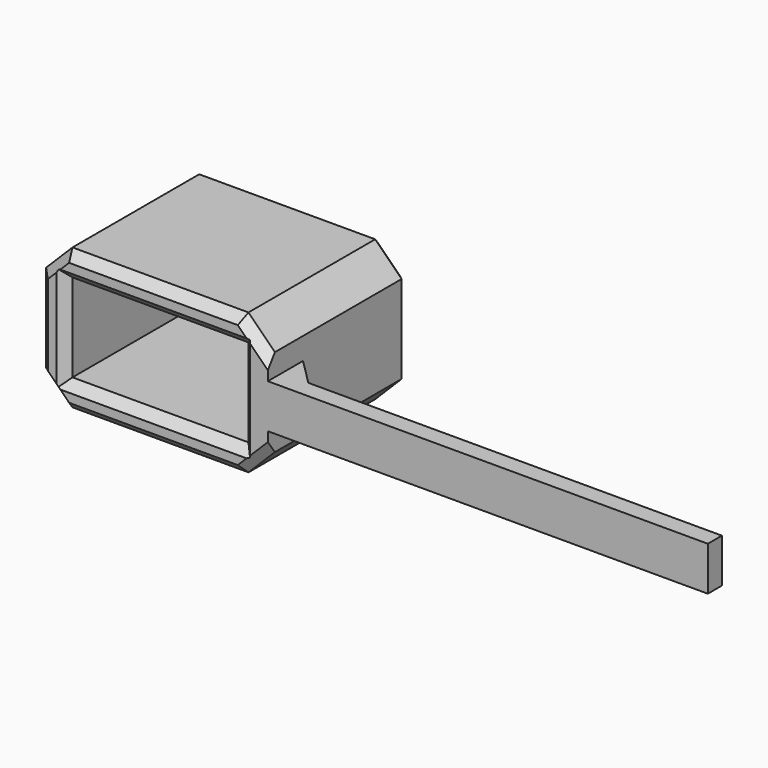
from build123d import *

# Parameters (mm, degrees)
F0_W         = 26
F0_H         = 16
F0_W_2       = 20
F0_H_2       = 10
F1_DEPTH     = 20
F3_DEPTH     = 50
F4_SIZE      = 3
F5_T1_DEPTH  = 10
F5_T3_DEPTH  = 20
F5_T5_DEPTH  = 9.3860066631
F5_T7_DEPTH  = 9.3860066631
F5_T9_DEPTH  = 9.3860066631
F5_T11_DEPTH = 9.3860066631
F5_T13_DEPTH = 25.1433659759
F5_T15_DEPTH = 15.1433659759
F5_T21_DEPTH = 22.571682988
F5_T25_DEPTH = 12.571682988
F5_T32_DEPTH = 22.571682988
F5_T36_DEPTH = 12.571682988
F5_T43_DEPTH = 12.571682988
F5_T47_DEPTH = 22.571682988
F5_T54_DEPTH = 22.571682988
F5_T58_DEPTH = 12.571682988
F6_T1_DEPTH  = 9.3860066631
F6_T3_DEPTH  = 10
F6_T5_DEPTH  = 9.3860066631
F6_T7_DEPTH  = 25.1433659759
F6_T9_DEPTH  = 20
F6_T14_DEPTH = 9.3860066631
F6_T19_DEPTH = 9.3860066631
F6_T25_DEPTH = 22.571682988
F6_T30_DEPTH = 12.571682988
F6_T38_DEPTH = 22.571682988
F6_T43_DEPTH = 12.571682988
F6_T51_DEPTH = 22.571682988
F6_T56_DEPTH = 12.571682988
F6_T64_DEPTH = 12.571682988
F6_T69_DEPTH = 22.571682988
F7_SIZE      = 1


# Not quite as in the source:
# - a fillet or chamfer that OpenCascade refuses, or shapes differently, is made with other operations: its cross-section is extruded or revolved along the edge and cut away or added


with BuildPart() as f1:
    # F0 (on Front) → F1 (new body)
    with BuildSketch(Plane.XZ):
        with Locations((10, 5)):
            Rectangle(F0_W, F0_H)
        with Locations((10, 5)):
            Rectangle(F0_W_2, F0_H_2, mode=Mode.SUBTRACT)
    extrude(amount=F1_DEPTH)

    # F2 (on face) → F3 (join)
    with BuildSketch(Plane.YZ.offset(23)):
        Polygon((-18, 2.5), (-18, 5), (-18, 7.5), (-20, 7.5), (-20, 5), (-20, 2.5), align=None)
    extrude(amount=F3_DEPTH)

    # F4
    f4_edges = [f1.edges().sort_by_distance(p)[0] for p in [
        (-3, -10, 13),
        (23, -10, 13),
        (23, -18, 5),
        (-3, -10, -3),
        (23, -10, -3),
    ]]
    chamfer(f4_edges, length=F4_SIZE)

    # F5: chamfer of 1 on 12 edges, made by hand

    # F5_s2 → F5_t1 (cut)
    with BuildSketch(Plane.XY):
        Polygon((21, 0), (20, -1), (20, 0), align=None)
        Polygon((-1, 0), (0, -1), (0, 0), align=None)
    extrude(amount=F5_T1_DEPTH, mode=Mode.SUBTRACT)

    # F5_s4 → F5_t3 (cut)
    with BuildSketch(Plane.YZ):
        Polygon((0, 11), (-1, 10), (0, 10), align=None)
        Polygon((0, -1), (-1, 0), (0, 0), align=None)
    extrude(amount=F5_T3_DEPTH, mode=Mode.SUBTRACT)

    # F5_s6 → F5_t5 (cut)
    with BuildSketch(Plane(origin=(-3.3184544799, 0, 3.3184544799), x_dir=(0, 1, 0), z_dir=(0.7071067812, 0, -0.7071067812))):
        Polygon((0, -1.1213203436), (-1, -2.1213203436), (0, -2.1213203436), align=None)
    extrude(amount=F5_T5_DEPTH, mode=Mode.SUBTRACT)

    # F5_s8 → F5_t7 (cut)
    with BuildSketch(Plane(origin=(13.3184544799, 0, 13.3184544799), x_dir=(0, 1, 0), z_dir=(-0.7071067812, 0, -0.7071067812))):
        Polygon((0, 15.2634559673), (-1, 16.2634559673), (0, 16.2634559673), align=None)
    extrude(amount=F5_T7_DEPTH, mode=Mode.SUBTRACT)

    # F5_s10 → F5_t9 (cut)
    with BuildSketch(Plane(origin=(1.6815455201, 0, -1.6815455201), x_dir=(0, 1, 0), z_dir=(0.7071067812, 0, -0.7071067812))):
        Polygon((0, 22.3345237792), (-1, 23.3345237792), (0, 23.3345237792), align=None)
    extrude(amount=F5_T9_DEPTH, mode=Mode.SUBTRACT)

    # F5_s12 → F5_t11 (cut)
    with BuildSketch(Plane(origin=(8.3184544799, 0, 8.3184544799), x_dir=(0, 1, 0), z_dir=(-0.7071067812, 0, -0.7071067812))):
        Polygon((0, -8.1923881554), (-1, -9.1923881554), (0, -9.1923881554), align=None)
    extrude(amount=F5_T11_DEPTH, mode=Mode.SUBTRACT)

    # F5_s14 → F5_t13 (cut)
    with BuildSketch(Plane.YZ.offset(-2.571682988)):
        Polygon((0, -2), (-1, -3), (0, -3), align=None)
        Polygon((-1, 13), (0, 12), (0, 13), align=None)
    extrude(amount=F5_T13_DEPTH, mode=Mode.SUBTRACT)

    # F5_s16 → F5_t15 (cut)
    with BuildSketch(Plane.XY.offset(-2.571682988)):
        Polygon((22, 0), (23, -1), (23, 0), align=None)
        Polygon((-2, 0), (-3, -1), (-3, 0), align=None)
    extrude(amount=F5_T15_DEPTH, mode=Mode.SUBTRACT)


with BuildPart() as f5_tool19:
    # F5_s20 → F5_t21 (new body)
    with BuildSketch(Plane.YZ):
        Polygon((0, 11), (-1, 10), (0, 10), align=None)
    extrude(amount=F5_T21_DEPTH)

    split(bisect_by=Plane.YZ.offset(20), keep=Keep.TOP)


with BuildPart() as f5_tool23:
    # F5_s24 → F5_t25 (new body)
    with BuildSketch(Plane.XY.offset(12.571682988)):
        Polygon((21, 0), (20, -1), (20, 0), align=None)
    extrude(amount=-F5_T25_DEPTH)

    split(bisect_by=Plane.XY.offset(10), keep=Keep.TOP)


with BuildPart() as f5_tool19_1:
    add(f5_tool19.part)

    # F5_t27: intersect F5_tool23
    add(f5_tool23.part, mode=Mode.INTERSECT)


with BuildPart() as f1_1:
    add(f1.part)

    # F5_t17: cut F5_tool19
    add(f5_tool19_1.part, mode=Mode.SUBTRACT)


with BuildPart() as f5_tool30:
    # F5_s31 → F5_t32 (new body)
    with BuildSketch(Plane.YZ.offset(22.571682988)):
        Polygon((0, -1), (-1, 0), (0, 0), align=None)
    extrude(amount=-F5_T32_DEPTH)

    split(bisect_by=Plane.YZ.offset(20), keep=Keep.TOP)


with BuildPart() as f5_tool34:
    # F5_s35 → F5_t36 (new body)
    with BuildSketch(Plane.XY.offset(10)):
        Polygon((21, 0), (20, -1), (20, 0), align=None)
    extrude(amount=-F5_T36_DEPTH)

    split(bisect_by=Plane.XY, keep=Keep.BOTTOM)


with BuildPart() as f5_tool30_1:
    add(f5_tool30.part)

    # F5_t38: intersect F5_tool34
    add(f5_tool34.part, mode=Mode.INTERSECT)


with BuildPart() as f1_2:
    add(f1_1.part)

    # F5_t28: cut F5_tool30
    add(f5_tool30_1.part, mode=Mode.SUBTRACT)


with BuildPart() as f5_tool41:
    # F5_s42 → F5_t43 (new body)
    with BuildSketch(Plane.XY):
        Polygon((-1, 0), (0, -1), (0, 0), align=None)
    extrude(amount=F5_T43_DEPTH)

    split(bisect_by=Plane.XY.offset(10), keep=Keep.TOP)


with BuildPart() as f5_tool45:
    # F5_s46 → F5_t47 (new body)
    with BuildSketch(Plane.YZ.offset(-2.571682988)):
        Polygon((0, 11), (-1, 10), (0, 10), align=None)
    extrude(amount=F5_T47_DEPTH)

    split(bisect_by=Plane.YZ, keep=Keep.BOTTOM)


with BuildPart() as f5_tool41_1:
    add(f5_tool41.part)

    # F5_t49: intersect F5_tool45
    add(f5_tool45.part, mode=Mode.INTERSECT)


with BuildPart() as f1_3:
    add(f1_2.part)

    # F5_t39: cut F5_tool41
    add(f5_tool41_1.part, mode=Mode.SUBTRACT)


with BuildPart() as f5_tool52:
    # F5_s53 → F5_t54 (new body)
    with BuildSketch(Plane.YZ.offset(20)):
        Polygon((0, -1), (-1, 0), (0, 0), align=None)
    extrude(amount=-F5_T54_DEPTH)

    split(bisect_by=Plane.YZ, keep=Keep.BOTTOM)


with BuildPart() as f5_tool56:
    # F5_s57 → F5_t58 (new body)
    with BuildSketch(Plane.XY.offset(-2.571682988)):
        Polygon((-1, 0), (0, -1), (0, 0), align=None)
    extrude(amount=F5_T58_DEPTH)

    split(bisect_by=Plane.XY, keep=Keep.BOTTOM)


with BuildPart() as f5_tool52_1:
    add(f5_tool52.part)

    # F5_t60: intersect F5_tool56
    add(f5_tool56.part, mode=Mode.INTERSECT)


with BuildPart() as f1_4:
    add(f1_3.part)

    # F5_t50: cut F5_tool52
    add(f5_tool52_1.part, mode=Mode.SUBTRACT)

    # F6: chamfer of 1 on 10 edges, made by hand

    # F6_s2 → F6_t1 (cut)
    with BuildSketch(Plane(origin=(-3.3184544799, 0, 3.3184544799), x_dir=(0, 1, 0), z_dir=(0.7071067812, 0, -0.7071067812))):
        Polygon((-19, -2.1213203436), (-20, -1.1213203436), (-20, -2.1213203436), align=None)
    extrude(amount=F6_T1_DEPTH, mode=Mode.SUBTRACT)

    # F6_s4 → F6_t3 (cut)
    with BuildSketch(Plane.XY):
        Polygon((0, -19), (-1, -20), (0, -20), align=None)
        Polygon((20, -19), (21, -20), (20, -20), align=None)
    extrude(amount=F6_T3_DEPTH, mode=Mode.SUBTRACT)

    # F6_s6 → F6_t5 (cut)
    with BuildSketch(Plane(origin=(8.3184544799, 0, 8.3184544799), x_dir=(0, 1, 0), z_dir=(-0.7071067812, 0, -0.7071067812))):
        Polygon((-20, -8.1923881554), (-19, -9.1923881554), (-20, -9.1923881554), align=None)
    extrude(amount=F6_T5_DEPTH, mode=Mode.SUBTRACT)

    # F6_s8 → F6_t7 (cut)
    with BuildSketch(Plane.YZ.offset(-2.571682988)):
        Polygon((-19, -3), (-20, -2), (-20, -3), align=None)
        Polygon((-19, 13), (-20, 12), (-20, 13), align=None)
    extrude(amount=F6_T7_DEPTH, mode=Mode.SUBTRACT)

    # F6_s10 → F6_t9 (cut)
    with BuildSketch(Plane.YZ):
        Polygon((-19, 0), (-20, -1), (-20, 0), align=None)
        Polygon((-19, 10), (-20, 11), (-20, 10), align=None)
    extrude(amount=F6_T9_DEPTH, mode=Mode.SUBTRACT)


with BuildPart() as f6_tool12:
    # F6_s13 → F6_t14 (new body)
    with BuildSketch(Plane(origin=(1.6815455201, 0, -1.6815455201), x_dir=(0, 1, 0), z_dir=(0.7071067812, 0, -0.7071067812))):
        Polygon((-19, 23.3345237792), (-20, 22.3345237792), (-20, 23.3345237792), align=None)
    extrude(amount=F6_T14_DEPTH)

    split(bisect_by=Plane.XY.offset(7.5), keep=Keep.TOP)


with BuildPart() as f1_5:
    add(f1_4.part)

    # F6_t11: cut F6_tool12
    add(f6_tool12.part, mode=Mode.SUBTRACT)


with BuildPart() as f6_tool17:
    # F6_s18 → F6_t19 (new body)
    with BuildSketch(Plane(origin=(13.3184544799, 0, 13.3184544799), x_dir=(0, 1, 0), z_dir=(-0.7071067812, 0, -0.7071067812))):
        Polygon((-19, 16.2634559673), (-20, 15.2634559673), (-20, 16.2634559673), align=None)
    extrude(amount=F6_T19_DEPTH)

    split(bisect_by=Plane.XY.offset(2.5), keep=Keep.BOTTOM)


with BuildPart() as f1_6:
    add(f1_5.part)

    # F6_t16: cut F6_tool17
    add(f6_tool17.part, mode=Mode.SUBTRACT)


with BuildPart() as f6_tool23:
    # F6_s24 → F6_t25 (new body)
    with BuildSketch(Plane.YZ.offset(20)):
        Polygon((-19, 0), (-20, -1), (-20, 0), align=None)
    extrude(amount=-F6_T25_DEPTH)

    split(bisect_by=Plane(origin=(-1.5, 0, -1.5), x_dir=(0, 1, 0), z_dir=(0.7071067812, 0, 0.7071067812)), keep=Keep.TOP)

    split(bisect_by=Plane.YZ, keep=Keep.BOTTOM)


with BuildPart() as f6_tool28:
    # F6_s29 → F6_t30 (new body)
    with BuildSketch(Plane.XY.offset(-2.571682988)):
        Polygon((0, -19), (-1, -20), (0, -20), align=None)
    extrude(amount=F6_T30_DEPTH)

    split(bisect_by=Plane(origin=(-1.5, 0, -1.5), x_dir=(0, 1, 0), z_dir=(0.7071067812, 0, 0.7071067812)), keep=Keep.TOP)

    split(bisect_by=Plane.XY, keep=Keep.BOTTOM)


with BuildPart() as f6_tool23_1:
    add(f6_tool23.part)

    # F6_t33: intersect F6_tool28
    add(f6_tool28.part, mode=Mode.INTERSECT)


with BuildPart() as f1_7:
    add(f1_6.part)

    # F6_t21: cut F6_tool23
    add(f6_tool23_1.part, mode=Mode.SUBTRACT)


with BuildPart() as f6_tool36:
    # F6_s37 → F6_t38 (new body)
    with BuildSketch(Plane.YZ.offset(-2.571682988)):
        Polygon((-19, 10), (-20, 11), (-20, 10), align=None)
    extrude(amount=F6_T38_DEPTH)

    split(bisect_by=Plane.YZ, keep=Keep.BOTTOM)

    split(bisect_by=Plane(origin=(-6.5, 0, 6.5), x_dir=(0, 1, 0), z_dir=(0.7071067812, 0, -0.7071067812)), keep=Keep.TOP)


with BuildPart() as f6_tool41:
    # F6_s42 → F6_t43 (new body)
    with BuildSketch(Plane.XY):
        Polygon((0, -19), (-1, -20), (0, -20), align=None)
    extrude(amount=F6_T43_DEPTH)

    split(bisect_by=Plane.XY.offset(10), keep=Keep.TOP)

    split(bisect_by=Plane(origin=(-6.5, 0, 6.5), x_dir=(0, 1, 0), z_dir=(0.7071067812, 0, -0.7071067812)), keep=Keep.TOP)


with BuildPart() as f6_tool36_1:
    add(f6_tool36.part)

    # F6_t46: intersect F6_tool41
    add(f6_tool41.part, mode=Mode.INTERSECT)


with BuildPart() as f1_8:
    add(f1_7.part)

    # F6_t34: cut F6_tool36
    add(f6_tool36_1.part, mode=Mode.SUBTRACT)


with BuildPart() as f6_tool49:
    # F6_s50 → F6_t51 (new body)
    with BuildSketch(Plane.YZ.offset(22.571682988)):
        Polygon((-19, 0), (-20, -1), (-20, 0), align=None)
    extrude(amount=-F6_T51_DEPTH)

    split(bisect_by=Plane(origin=(11.5, 0, -11.5), x_dir=(0, 1, 0), z_dir=(-0.7071067812, 0, 0.7071067812)), keep=Keep.TOP)

    split(bisect_by=Plane.YZ.offset(20), keep=Keep.TOP)


with BuildPart() as f6_tool54:
    # F6_s55 → F6_t56 (new body)
    with BuildSketch(Plane.XY.offset(10)):
        Polygon((20, -19), (21, -20), (20, -20), align=None)
    extrude(amount=-F6_T56_DEPTH)

    split(bisect_by=Plane(origin=(11.5, 0, -11.5), x_dir=(0, 1, 0), z_dir=(-0.7071067812, 0, 0.7071067812)), keep=Keep.TOP)

    split(bisect_by=Plane.XY, keep=Keep.BOTTOM)


with BuildPart() as f6_tool49_1:
    add(f6_tool49.part)

    # F6_t59: intersect F6_tool54
    add(f6_tool54.part, mode=Mode.INTERSECT)


with BuildPart() as f1_9:
    add(f1_8.part)

    # F6_t47: cut F6_tool49
    add(f6_tool49_1.part, mode=Mode.SUBTRACT)


with BuildPart() as f6_tool62:
    # F6_s63 → F6_t64 (new body)
    with BuildSketch(Plane.XY.offset(12.571682988)):
        Polygon((20, -19), (21, -20), (20, -20), align=None)
    extrude(amount=-F6_T64_DEPTH)

    split(bisect_by=Plane(origin=(16.5, 0, 16.5), x_dir=(0, 1, 0), z_dir=(-0.7071067812, 0, -0.7071067812)), keep=Keep.TOP)

    split(bisect_by=Plane.XY.offset(10), keep=Keep.TOP)


with BuildPart() as f6_tool67:
    # F6_s68 → F6_t69 (new body)
    with BuildSketch(Plane.YZ):
        Polygon((-19, 10), (-20, 11), (-20, 10), align=None)
    extrude(amount=F6_T69_DEPTH)

    split(bisect_by=Plane(origin=(16.5, 0, 16.5), x_dir=(0, 1, 0), z_dir=(-0.7071067812, 0, -0.7071067812)), keep=Keep.TOP)

    split(bisect_by=Plane.YZ.offset(20), keep=Keep.TOP)


with BuildPart() as f6_tool62_1:
    add(f6_tool62.part)

    # F6_t72: intersect F6_tool67
    add(f6_tool67.part, mode=Mode.INTERSECT)


with BuildPart() as f1_10:
    add(f1_9.part)

    # F6_t60: cut F6_tool62
    add(f6_tool62_1.part, mode=Mode.SUBTRACT)

    # F7
    f7_edges = [f1_10.edges().sort_by_distance(p)[0] for p in [
        (-3, -20, 5),
    ]]
    chamfer(f7_edges, length=F7_SIZE)


solid = f1_10.part
